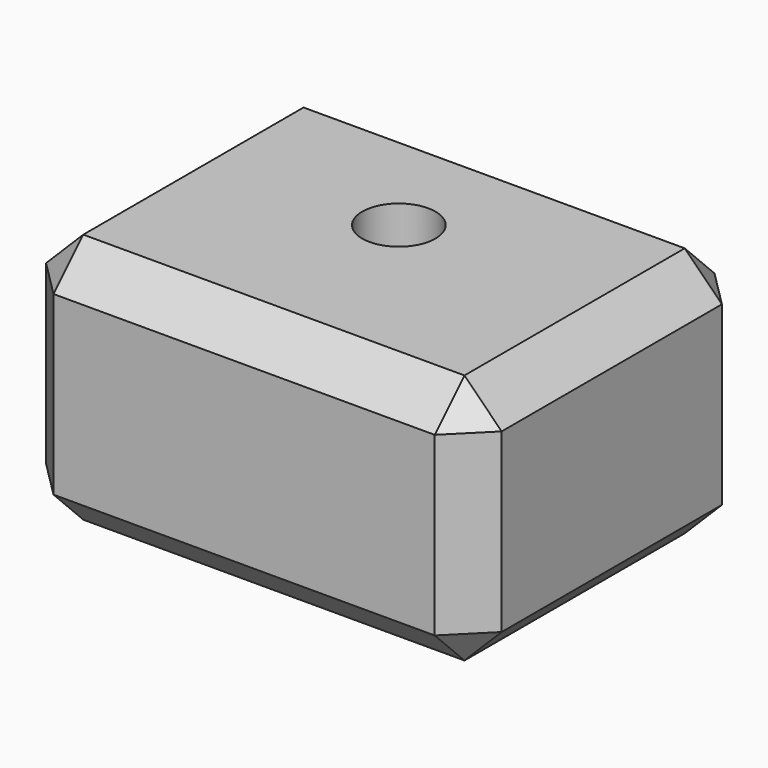
from build123d import *

# Parameters (mm, degrees)
F0_W     = 62.2431822121
F0_H     = 47.7795563638
F1_DEPTH = 34.29
F2_SIZE  = 5.08
F4_D     = 10


with BuildPart() as f1:
    # F0 (on Top) → F1 (new body)
    with BuildSketch(Plane.XY):
        with Locations((-85.0962679833, -23.8897781819)):
            Rectangle(F0_W, F0_H)
    extrude(amount=F1_DEPTH)

    # F2
    f2_edges = [f1.edges().sort_by_distance(p)[0] for p in [
        (-116.217859, -47.779556, 17.145),
        (-53.974677, -47.779556, 17.145),
        (-85.096268, -47.779556, 0),
        (-85.096268, -47.779556, 34.29),
        (-85.096268, 0, 34.29),
        (-116.217859, -23.889778, 34.29),
        (-53.974677, -23.889778, 34.29),
        (-53.974677, 0, 17.145),
        (-53.974677, -23.889778, 0),
        (-116.217859, 0, 17.145),
        (-116.217859, -23.889778, 0),
        (-85.096268, 0, 0),
    ]]
    chamfer(f2_edges, length=F2_SIZE)

    # F4 (through all)
    with Locations(Plane.XY.offset(34.29)):
        with Locations((-86.2206369638, -19.9478901923)):
            Hole(F4_D / 2)


solid = f1.part
